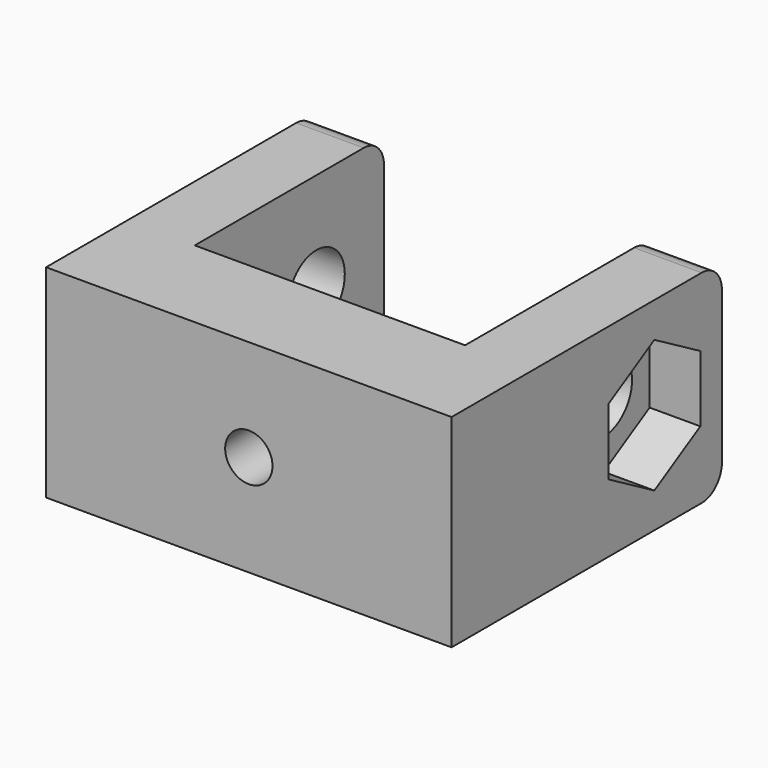
from build123d import *

# Parameters (mm, degrees)
F1_DEPTH  = 6
F2_R      = 2.1
F3_DEPTH  = 25
F6_DEPTH  = 3
F7_R      = 1.5
F9_R      = 1.4
F10_DEPTH = 5


with BuildPart() as f1:
    # F0 (on Top) → F1 (new body, symmetric)
    with BuildSketch(Plane.XY):
        Polygon((12, -10), (12, 10), (8, 10), (8, -4), (0, -4), (-8, -4), (-8, 10), (-12, 10), (-12, -10), align=None)
    extrude(amount=F1_DEPTH, both=True)

    # F2 (on Right) → F3 (cut, symmetric)
    with BuildSketch(Plane.YZ):
        with Locations((5, 0)):
            Circle(F2_R)
    extrude(amount=F3_DEPTH, both=True, mode=Mode.SUBTRACT)

    # F5 (on offset) → F6 (cut)
    with BuildSketch(Plane.YZ.offset(12)):
        Polygon((5, -3.9259818305), (8.4, -1.9629909152), (8.4, 1.9629909152), (5, 3.9259818305), (1.6, 1.9629909152), (1.6, -1.9629909152), align=None)
    extrude(amount=-F6_DEPTH, mode=Mode.SUBTRACT)

    # F7
    f7_edges = [f1.edges().sort_by_distance(p)[0] for p in [
        (10, 10, -6),
        (10, 10, 6),
        (-10, 10, -6),
        (-10, 10, 6),
    ]]
    fillet(f7_edges, radius=F7_R)

    # F9 (on offset) → F10 (cut)
    with BuildSketch(Plane.XZ.offset(10)):
        Circle(F9_R)
    extrude(amount=-F10_DEPTH, mode=Mode.SUBTRACT)


solid = f1.part
